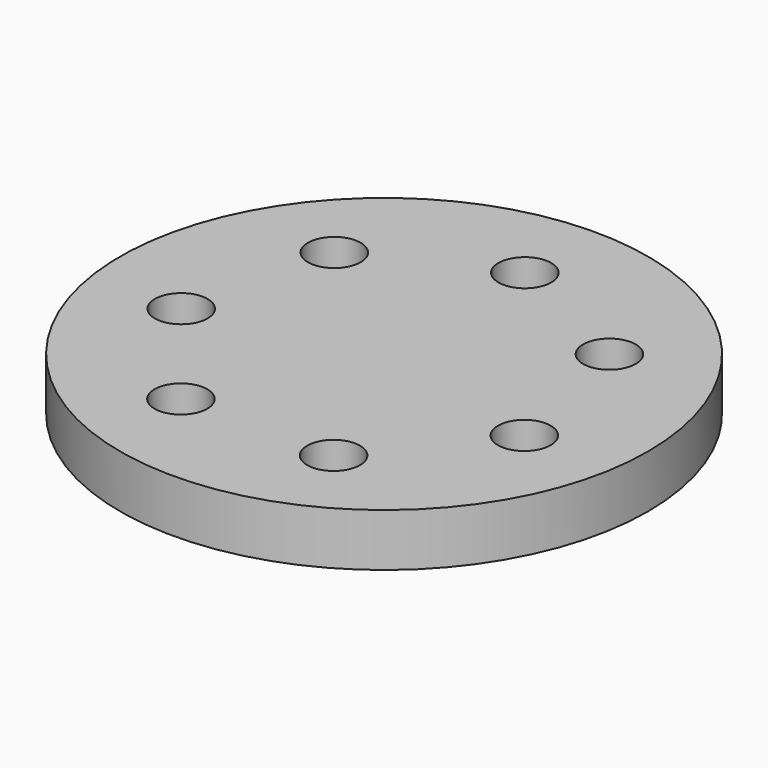
from build123d import *

# Parameters (mm, degrees)
F2_R            = 65
F3_DEPTH        = 13
F4_R            = 6.5
F5_DEPTH        = 13.001
F5_COPIES_COUNT = 7


# Not quite as in the source:
# - a pattern or mirror of a feature is missing from the dataset's text; its kind, count and spacing are read off the source's solid


with BuildPart() as f3:
    # F2 (on Top) → F3 (new body)
    with BuildSketch(Plane.XY):
        Circle(F2_R)
    extrude(amount=F3_DEPTH)

    # F4 (on face) → F5 (cut, through all)
    with BuildSketch(Plane.XY.offset(13)):
        with Locations((0, 43.3333333333)):
            Circle(F4_R)
    f5 = extrude(amount=-F5_DEPTH, mode=Mode.SUBTRACT)

    # F5_copies: F5 ×7 about axis
    f5_copies_axis = Axis((0, 0, 0), (0, 0, 1))
    for i in range(1, F5_COPIES_COUNT):
        add(f5.rotate(f5_copies_axis, i * 360 / F5_COPIES_COUNT), mode=Mode.SUBTRACT)


solid = f3.part
